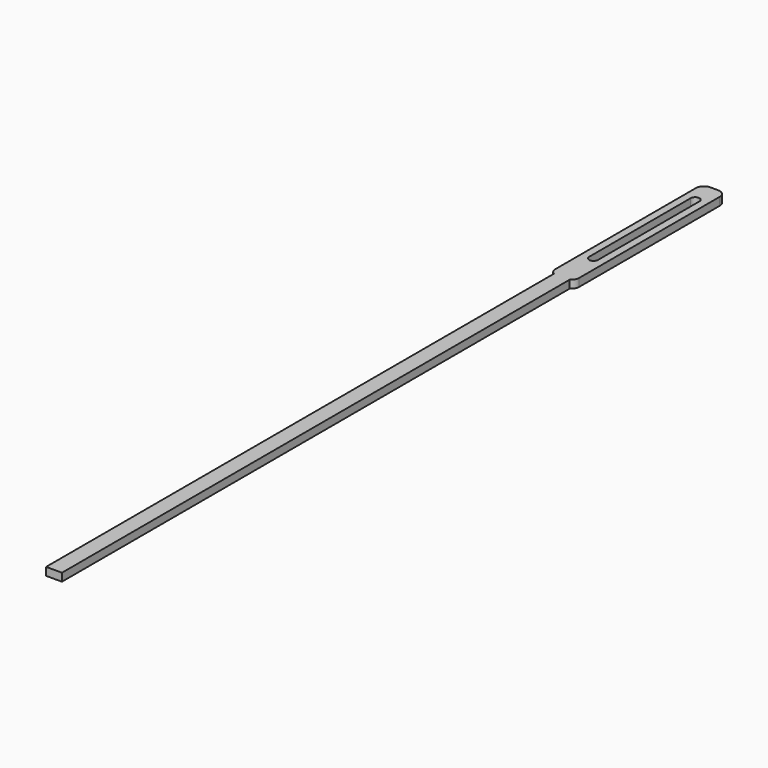
from build123d import *

# Parameters (mm, degrees)
F1_DEPTH    = 6.35
F2_T1_DEPTH = 38.1
F2_T3_DEPTH = 33.8463065702
F4_DEPTH    = 6.351


# Not quite as in the source:
# - a fillet or chamfer that OpenCascade refuses, or shapes differently, is made with other operations: its cross-section is extruded or revolved along the edge and cut away or added


with BuildPart() as f1:
    # F0 (on Top) → F1 (new body)
    with BuildSketch(Plane.XY):
        Polygon((-3.1513119073, 592.2723904558), (-22.2013119073, 592.2723904558), (-22.2013119073, 439.8723904558), (-19.0263119073, 439.8723904558), (-19.0263119073, -68.1276095442), (-6.3263119073, -68.1276095442), (-6.3263119073, 439.8723904558), (-3.1513119073, 439.8723904558), align=None)
    extrude(amount=F1_DEPTH)

    # F2: fillet of radius 6.35 on 4 edges, made by hand

    # F2_s2 → F2_t1 (cut)
    with BuildSketch(Plane.XY.offset(-15.875)):
        with BuildLine():
            ThreePointArc((-3.1513119073, 585.9223904558), (-5.0111838468, 590.4125185164), (-9.5013119073, 592.2723904558))
            Line((-9.5013119073, 592.2723904558), (-3.1513119073, 592.2723904558))
            Line((-3.1513119073, 592.2723904558), (-3.1513119073, 585.9223904558))
        make_face()
        with BuildLine():
            ThreePointArc((-15.8513119073, 592.2723904558), (-20.3414399678, 590.4125185164), (-22.2013119073, 585.9223904558))
            Line((-22.2013119073, 585.9223904558), (-22.2013119073, 592.2723904558))
            Line((-22.2013119073, 592.2723904558), (-15.8513119073, 592.2723904558))
        make_face()
    extrude(amount=F2_T1_DEPTH, mode=Mode.SUBTRACT)

    # F2_s4 → F2_t3 (cut)
    with BuildSketch(Plane.XY.offset(-13.7481532851)):
        with BuildLine():
            ThreePointArc((-22.2013119073, 445.3716517699), (-21.3505732213, 442.1966517699), (-19.0263119073, 439.8723904558))
            Line((-19.0263119073, 439.8723904558), (-22.2013119073, 439.8723904558))
            Line((-22.2013119073, 439.8723904558), (-22.2013119073, 445.3716517699))
        make_face()
        with BuildLine():
            ThreePointArc((-6.3263119073, 439.8723904558), (-4.0020505933, 442.1966517699), (-3.1513119073, 445.3716517699))
            Line((-3.1513119073, 445.3716517699), (-3.1513119073, 439.8723904558))
            Line((-3.1513119073, 439.8723904558), (-6.3263119073, 439.8723904558))
        make_face()
    extrude(amount=F2_T3_DEPTH, mode=Mode.SUBTRACT)

    # F3 (on face) → F4 (cut, through all)
    with BuildSketch(Plane(origin=(0, 0, 0), x_dir=(1, 0, 0), z_dir=(0, 0, -1))):
        with BuildLine():
            Line((-16.1688119073, -471.6223904558), (-16.1688119073, -573.2223904558))
            ThreePointArc((-16.1688119073, -573.2223904558), (-12.6763119073, -576.7148904558), (-9.1838119073, -573.2223904558))
            Line((-9.1838119073, -573.2223904558), (-9.1838119073, -471.6223904558))
            ThreePointArc((-9.1838119073, -471.6223904558), (-12.6763119073, -468.1298904558), (-16.1688119073, -471.6223904558))
        make_face()
    extrude(amount=-F4_DEPTH, mode=Mode.SUBTRACT)


solid = f1.part
